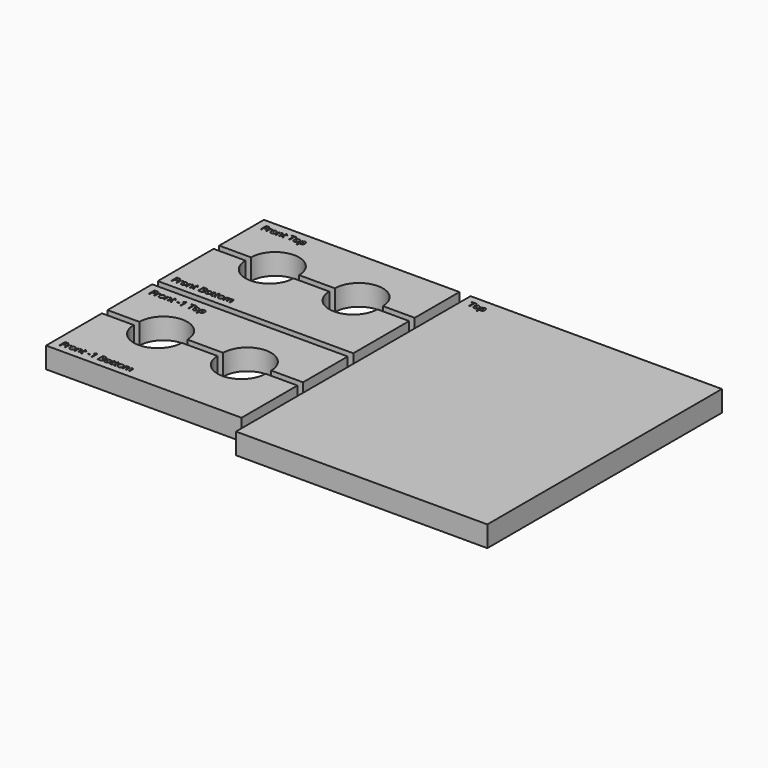
from build123d import *

# Parameters (mm, degrees)
F1_DEPTH = 9.525
F0_W     = 1.0569552951
F0_H     = 0.3272840712
F0_W_2   = 114.3
F0_H_2   = 133.35


# Not quite as in the source:
# - a length typed as a fraction of an inch, garbled in the dataset ("3 / 203.2 mm" for 3/8 in), is restored


with BuildPart() as f1:
    # F0 (on Top) → F1 (new body)
    with BuildSketch(Plane.XY):
        with BuildLine():
            Line((44.45, 0), (-44.45, 0))
            Line((-44.45, 0), (-44.45, -25.4))
            Line((-44.45, -25.4), (-29.972, -25.4))
            ThreePointArc((-29.972, -25.4), (-19.05, -14.478), (-8.128, -25.4))
            Line((-8.128, -25.4), (8.128, -25.4))
            ThreePointArc((8.128, -25.4), (19.05, -14.478), (29.972, -25.4))
            Line((29.972, -25.4), (44.45, -25.4))
            Line((44.45, -25.4), (44.45, 0))
        make_face()
        Polygon((-40.4764268663, -5.0043457031), (-40.4764268663, -6.35), (-40.8422960069, -6.35), (-40.8422960069, -3.2018717448), (-39.0873643663, -3.2018717448), (-39.0873643663, -3.5270887587), (-40.4764268663, -3.5270887587), (-40.4764268663, -4.6791286892), (-39.1714246962, -4.6791286892), (-39.1714246962, -5.0043457031), align=None, mode=Mode.SUBTRACT)
        with BuildLine():
            add(Edge.make_bspline(
                [(-37.9504828559, -4.071758355), (-37.7651367187, -3.9467013889), (-37.5432725694, -3.9467013889)],
                knots=[0, 0, 0, 1, 1, 1], degree=2))
            add(Edge.make_bspline(
                [(-37.5432725694, -3.9467013889), (-37.3861762153, -3.9467013889), (-37.2614637587, -3.9728841146)],
                knots=[0, 0, 0, 1, 1, 1], degree=2))
            Line((-37.2614637587, -3.9728841146), (-37.3110731337, -4.3043023003))
            add(Edge.make_bspline(
                [(-37.3110731337, -4.3043023003), (-37.4571451823, -4.2719184028), (-37.5694552951, -4.2719184028)],
                knots=[0, 0, 0, 1, 1, 1], degree=2))
            add(Edge.make_bspline(
                [(-37.5694552951, -4.2719184028), (-37.8560872396, -4.2719184028), (-38.0593478733, -4.5044623481)],
                knots=[0, 0, 0, 1, 1, 1], degree=2))
            add(Edge.make_bspline(
                [(-38.0593478733, -4.5044623481), (-38.2626085069, -4.7370062934), (-38.2626085069, -5.0835828993)],
                knots=[0, 0, 0, 1, 1, 1], degree=2))
            Line((-38.2626085069, -5.0835828993), (-38.2626085069, -6.35))
            Line((-38.2626085069, -6.35), (-38.6202094184, -6.35))
            Line((-38.6202094184, -6.35), (-38.6202094184, -3.990109592))
            Line((-38.6202094184, -3.990109592), (-38.3253092448, -3.990109592))
            Line((-38.3253092448, -3.990109592), (-38.283968099, -4.4269476997))
            Line((-38.283968099, -4.4269476997), (-38.2667426215, -4.4269476997))
            add(Edge.make_bspline(
                [(-38.2667426215, -4.4269476997), (-38.1358289931, -4.1968153212), (-37.9504828559, -4.071758355)],
                knots=[0, 0, 0, 1, 1, 1], degree=2))
        make_face(mode=Mode.SUBTRACT)
        with BuildLine():
            add(Edge.make_bspline(
                [(-35.0748616536, -4.2763970269), (-34.783062066, -4.6060926649), (-34.783062066, -5.1676432292)],
                knots=[0, 0, 0, 1, 1, 1], degree=2))
            add(Edge.make_bspline(
                [(-34.783062066, -5.1676432292), (-34.783062066, -5.7450412326), (-35.0734836155, -6.0692247179)],
                knots=[0, 0, 0, 1, 1, 1], degree=2))
            add(Edge.make_bspline(
                [(-35.0734836155, -6.0692247179), (-35.3639051649, -6.3934082031), (-35.8765353733, -6.3934082031)],
                knots=[0, 0, 0, 1, 1, 1], degree=2))
            add(Edge.make_bspline(
                [(-35.8765353733, -6.3934082031), (-36.193484158, -6.3934082031), (-36.4387749566, -6.2445800781)],
                knots=[0, 0, 0, 1, 1, 1], degree=2))
            add(Edge.make_bspline(
                [(-36.4387749566, -6.2445800781), (-36.6840657552, -6.0957519531), (-36.8177354601, -5.8180772569)],
                knots=[0, 0, 0, 1, 1, 1], degree=2))
            add(Edge.make_bspline(
                [(-36.8177354601, -5.8180772569), (-36.9514051649, -5.5404025608), (-36.9514051649, -5.1676432292)],
                knots=[0, 0, 0, 1, 1, 1], degree=2))
            add(Edge.make_bspline(
                [(-36.9514051649, -5.1676432292), (-36.9514051649, -4.5909342448), (-36.6627061632, -4.2688178168)],
                knots=[0, 0, 0, 1, 1, 1], degree=2))
            add(Edge.make_bspline(
                [(-36.6627061632, -4.2688178168), (-36.3740071615, -3.9467013889), (-35.8613769531, -3.9467013889)],
                knots=[0, 0, 0, 1, 1, 1], degree=2))
            add(Edge.make_bspline(
                [(-35.8613769531, -3.9467013889), (-35.3666612413, -3.9467013889), (-35.0748616536, -4.2763970269)],
                knots=[0, 0, 0, 1, 1, 1], degree=2))
        make_face(mode=Mode.SUBTRACT)
        with BuildLine():
            Line((-32.1833930122, -6.35), (-32.5409939236, -6.35))
            Line((-32.5409939236, -6.35), (-32.5409939236, -4.8231336806))
            add(Edge.make_bspline(
                [(-32.5409939236, -4.8231336806), (-32.5409939236, -4.5351236979), (-32.6722520616, -4.3928412543)],
                knots=[0, 0, 0, 1, 1, 1], degree=2))
            add(Edge.make_bspline(
                [(-32.6722520616, -4.3928412543), (-32.8035101997, -4.2505588108), (-33.0839409722, -4.2505588108)],
                knots=[0, 0, 0, 1, 1, 1], degree=2))
            add(Edge.make_bspline(
                [(-33.0839409722, -4.2505588108), (-33.4539442274, -4.2505588108), (-33.6261990017, -4.4507188585)],
                knots=[0, 0, 0, 1, 1, 1], degree=2))
            add(Edge.make_bspline(
                [(-33.6261990017, -4.4507188585), (-33.798453776, -4.6508789062), (-33.798453776, -5.1118326823)],
                knots=[0, 0, 0, 1, 1, 1], degree=2))
            Line((-33.798453776, -5.1118326823), (-33.798453776, -6.35))
            Line((-33.798453776, -6.35), (-34.1560546875, -6.35))
            Line((-34.1560546875, -6.35), (-34.1560546875, -3.990109592))
            Line((-34.1560546875, -3.990109592), (-33.8652886285, -3.990109592))
            Line((-33.8652886285, -3.990109592), (-33.8074110243, -4.3132595486))
            Line((-33.8074110243, -4.3132595486), (-33.7901855469, -4.3132595486))
            add(Edge.make_bspline(
                [(-33.7901855469, -4.3132595486), (-33.6799424913, -4.138937717), (-33.4818495009, -4.042819553)],
                knots=[0, 0, 0, 1, 1, 1], degree=2))
            add(Edge.make_bspline(
                [(-33.4818495009, -4.042819553), (-33.2837565104, -3.9467013889), (-33.0405327691, -3.9467013889)],
                knots=[0, 0, 0, 1, 1, 1], degree=2))
            add(Edge.make_bspline(
                [(-33.0405327691, -3.9467013889), (-32.6140299479, -3.9467013889), (-32.39871148, -4.1523735894)],
                knots=[0, 0, 0, 1, 1, 1], degree=2))
            add(Edge.make_bspline(
                [(-32.39871148, -4.1523735894), (-32.1833930122, -4.3580457899), (-32.1833930122, -4.8107313368)],
                knots=[0, 0, 0, 1, 1, 1], degree=2))
            Line((-32.1833930122, -4.8107313368), (-32.1833930122, -6.35))
        make_face(mode=Mode.SUBTRACT)
        with BuildLine():
            add(Edge.make_bspline(
                [(-30.9652072483, -5.9837863498), (-30.863921441, -6.0978190104), (-30.6875325521, -6.0978190104)],
                knots=[0, 0, 0, 1, 1, 1], degree=2))
            add(Edge.make_bspline(
                [(-30.6875325521, -6.0978190104), (-30.5924479167, -6.0978190104), (-30.5042534722, -6.0840386285)],
                knots=[0, 0, 0, 1, 1, 1], degree=2))
            add(Edge.make_bspline(
                [(-30.5042534722, -6.0840386285), (-30.4160590278, -6.0702582465), (-30.3643825955, -6.0550998264)],
                knots=[0, 0, 0, 1, 1, 1], degree=2))
            Line((-30.3643825955, -6.0550998264), (-30.3643825955, -6.328640408))
            add(Edge.make_bspline(
                [(-30.3643825955, -6.328640408), (-30.4222601997, -6.3562011719), (-30.5352593316, -6.3748046875)],
                knots=[0, 0, 0, 1, 1, 1], degree=2))
            add(Edge.make_bspline(
                [(-30.5352593316, -6.3748046875), (-30.6482584635, -6.3934082031), (-30.7392089844, -6.3934082031)],
                knots=[0, 0, 0, 1, 1, 1], degree=2))
            add(Edge.make_bspline(
                [(-30.7392089844, -6.3934082031), (-31.4234049479, -6.3934082031), (-31.4234049479, -5.6720052083)],
                knots=[0, 0, 0, 1, 1, 1], degree=2))
            Line((-31.4234049479, -5.6720052083), (-31.4234049479, -4.2677842882))
            Line((-31.4234049479, -4.2677842882), (-31.7617133247, -4.2677842882))
            Line((-31.7617133247, -4.2677842882), (-31.7617133247, -4.0955295139))
            Line((-31.7617133247, -4.0955295139), (-31.4234049479, -3.9467013889))
            Line((-31.4234049479, -3.9467013889), (-31.2731987847, -3.4430284288))
            Line((-31.2731987847, -3.4430284288), (-31.0664930556, -3.4430284288))
            Line((-31.0664930556, -3.4430284288), (-31.0664930556, -3.990109592))
            Line((-31.0664930556, -3.990109592), (-30.3816080729, -3.990109592))
            Line((-30.3816080729, -3.990109592), (-30.3816080729, -4.2677842882))
            Line((-30.3816080729, -4.2677842882), (-31.0664930556, -4.2677842882))
            Line((-31.0664930556, -4.2677842882), (-31.0664930556, -5.6568467882))
            add(Edge.make_bspline(
                [(-31.0664930556, -5.6568467882), (-31.0664930556, -5.8697536892), (-30.9652072483, -5.9837863498)],
                knots=[0, 0, 0, 1, 1, 1], degree=2))
        make_face(mode=Mode.SUBTRACT)
        Polygon((-27.724750434, -3.5270887587), (-27.724750434, -6.35), (-28.0906195747, -6.35), (-28.0906195747, -3.5270887587), (-29.0876302083, -3.5270887587), (-29.0876302083, -3.2018717448), (-26.7277398003, -3.2018717448), (-26.7277398003, -3.5270887587), align=None, mode=Mode.SUBTRACT)
        with BuildLine():
            add(Edge.make_bspline(
                [(-24.5624972873, -4.2763970269), (-24.2706976997, -4.6060926649), (-24.2706976997, -5.1676432292)],
                knots=[0, 0, 0, 1, 1, 1], degree=2))
            add(Edge.make_bspline(
                [(-24.2706976997, -5.1676432292), (-24.2706976997, -5.7450412326), (-24.5611192491, -6.0692247179)],
                knots=[0, 0, 0, 1, 1, 1], degree=2))
            add(Edge.make_bspline(
                [(-24.5611192491, -6.0692247179), (-24.8515407986, -6.3934082031), (-25.3641710069, -6.3934082031)],
                knots=[0, 0, 0, 1, 1, 1], degree=2))
            add(Edge.make_bspline(
                [(-25.3641710069, -6.3934082031), (-25.6811197917, -6.3934082031), (-25.9264105903, -6.2445800781)],
                knots=[0, 0, 0, 1, 1, 1], degree=2))
            add(Edge.make_bspline(
                [(-25.9264105903, -6.2445800781), (-26.1717013889, -6.0957519531), (-26.3053710937, -5.8180772569)],
                knots=[0, 0, 0, 1, 1, 1], degree=2))
            add(Edge.make_bspline(
                [(-26.3053710937, -5.8180772569), (-26.4390407986, -5.5404025608), (-26.4390407986, -5.1676432292)],
                knots=[0, 0, 0, 1, 1, 1], degree=2))
            add(Edge.make_bspline(
                [(-26.4390407986, -5.1676432292), (-26.4390407986, -4.5909342448), (-26.1503417969, -4.2688178168)],
                knots=[0, 0, 0, 1, 1, 1], degree=2))
            add(Edge.make_bspline(
                [(-26.1503417969, -4.2688178168), (-25.8616427951, -3.9467013889), (-25.3490125868, -3.9467013889)],
                knots=[0, 0, 0, 1, 1, 1], degree=2))
            add(Edge.make_bspline(
                [(-25.3490125868, -3.9467013889), (-24.854296875, -3.9467013889), (-24.5624972873, -4.2763970269)],
                knots=[0, 0, 0, 1, 1, 1], degree=2))
        make_face(mode=Mode.SUBTRACT)
        with BuildLine():
            add(Edge.make_bspline(
                [(-21.8250244141, -6.0712917752), (-22.0844401042, -6.3934082031), (-22.5453938802, -6.3934082031)],
                knots=[0, 0, 0, 1, 1, 1], degree=2))
            add(Edge.make_bspline(
                [(-22.5453938802, -6.3934082031), (-22.7762152778, -6.3934082031), (-22.9667290582, -6.3083143446)],
                knots=[0, 0, 0, 1, 1, 1], degree=2))
            add(Edge.make_bspline(
                [(-22.9667290582, -6.3083143446), (-23.1572428385, -6.2232204861), (-23.2860894097, -6.0461425781)],
                knots=[0, 0, 0, 1, 1, 1], degree=2))
            Line((-23.2860894097, -6.0461425781), (-23.3122721354, -6.0461425781))
            add(Edge.make_bspline(
                [(-23.3122721354, -6.0461425781), (-23.2860894097, -6.2528483073), (-23.2860894097, -6.4381944444)],
                knots=[0, 0, 0, 1, 1, 1], degree=2))
            Line((-23.2860894097, -6.4381944444), (-23.2860894097, -7.4097113715))
            Line((-23.2860894097, -7.4097113715), (-23.6436903212, -7.4097113715))
            Line((-23.6436903212, -7.4097113715), (-23.6436903212, -3.990109592))
            Line((-23.6436903212, -3.990109592), (-23.3529242622, -3.990109592))
            Line((-23.3529242622, -3.990109592), (-23.3033148872, -4.3132595486))
            Line((-23.3033148872, -4.3132595486), (-23.2860894097, -4.3132595486))
            add(Edge.make_bspline(
                [(-23.2860894097, -4.3132595486), (-23.1482855903, -4.1189561632), (-22.96535102, -4.032828776)],
                knots=[0, 0, 0, 1, 1, 1], degree=2))
            add(Edge.make_bspline(
                [(-22.96535102, -4.032828776), (-22.7824164497, -3.9467013889), (-22.5453938802, -3.9467013889)],
                knots=[0, 0, 0, 1, 1, 1], degree=2))
            add(Edge.make_bspline(
                [(-22.5453938802, -3.9467013889), (-22.076171875, -3.9467013889), (-21.8208902995, -4.2677842882)],
                knots=[0, 0, 0, 1, 1, 1], degree=2))
            add(Edge.make_bspline(
                [(-21.8208902995, -4.2677842882), (-21.565608724, -4.5888671875), (-21.565608724, -5.1676432292)],
                knots=[0, 0, 0, 1, 1, 1], degree=2))
            add(Edge.make_bspline(
                [(-21.565608724, -5.1676432292), (-21.565608724, -5.7491753472), (-21.8250244141, -6.0712917752)],
                knots=[0, 0, 0, 1, 1, 1], degree=2))
        make_face(mode=Mode.SUBTRACT)
    extrude(amount=F1_DEPTH)


with BuildPart() as f1b:
    # F0 (on Top) → F1, piece 2 (new body)
    with BuildSketch(Plane.XY):
        with BuildLine():
            Line((-29.972, -28.575), (-44.45, -28.575))
            Line((-44.45, -28.575), (-44.45, -60.325))
            Line((-44.45, -60.325), (44.45, -60.325))
            Line((44.45, -60.325), (44.45, -28.575))
            Line((44.45, -28.575), (29.972, -28.575))
            ThreePointArc((29.972, -28.575), (19.05, -39.497), (8.128, -28.575))
            Line((8.128, -28.575), (-8.128, -28.575))
            ThreePointArc((-8.128, -28.575), (-19.05, -39.497), (-29.972, -28.575))
        make_face()
        Polygon((-40.4764268663, -55.8043457031), (-40.4764268663, -57.15), (-40.8422960069, -57.15), (-40.8422960069, -54.0018717448), (-39.0873643663, -54.0018717448), (-39.0873643663, -54.3270887587), (-40.4764268663, -54.3270887587), (-40.4764268663, -55.4791286892), (-39.1714246962, -55.4791286892), (-39.1714246962, -55.8043457031), align=None, mode=Mode.SUBTRACT)
        with BuildLine():
            add(Edge.make_bspline(
                [(-37.9504828559, -54.871758355), (-37.7651367187, -54.7467013889), (-37.5432725694, -54.7467013889)],
                knots=[0, 0, 0, 1, 1, 1], degree=2))
            add(Edge.make_bspline(
                [(-37.5432725694, -54.7467013889), (-37.3861762153, -54.7467013889), (-37.2614637587, -54.7728841146)],
                knots=[0, 0, 0, 1, 1, 1], degree=2))
            Line((-37.2614637587, -54.7728841146), (-37.3110731337, -55.1043023003))
            add(Edge.make_bspline(
                [(-37.3110731337, -55.1043023003), (-37.4571451823, -55.0719184028), (-37.5694552951, -55.0719184028)],
                knots=[0, 0, 0, 1, 1, 1], degree=2))
            add(Edge.make_bspline(
                [(-37.5694552951, -55.0719184028), (-37.8560872396, -55.0719184028), (-38.0593478733, -55.3044623481)],
                knots=[0, 0, 0, 1, 1, 1], degree=2))
            add(Edge.make_bspline(
                [(-38.0593478733, -55.3044623481), (-38.2626085069, -55.5370062934), (-38.2626085069, -55.8835828993)],
                knots=[0, 0, 0, 1, 1, 1], degree=2))
            Line((-38.2626085069, -55.8835828993), (-38.2626085069, -57.15))
            Line((-38.2626085069, -57.15), (-38.6202094184, -57.15))
            Line((-38.6202094184, -57.15), (-38.6202094184, -54.790109592))
            Line((-38.6202094184, -54.790109592), (-38.3253092448, -54.790109592))
            Line((-38.3253092448, -54.790109592), (-38.283968099, -55.2269476997))
            Line((-38.283968099, -55.2269476997), (-38.2667426215, -55.2269476997))
            add(Edge.make_bspline(
                [(-38.2667426215, -55.2269476997), (-38.1358289931, -54.9968153212), (-37.9504828559, -54.871758355)],
                knots=[0, 0, 0, 1, 1, 1], degree=2))
        make_face(mode=Mode.SUBTRACT)
        with BuildLine():
            add(Edge.make_bspline(
                [(-35.0748616536, -55.0763970269), (-34.783062066, -55.4060926649), (-34.783062066, -55.9676432292)],
                knots=[0, 0, 0, 1, 1, 1], degree=2))
            add(Edge.make_bspline(
                [(-34.783062066, -55.9676432292), (-34.783062066, -56.5450412326), (-35.0734836155, -56.8692247179)],
                knots=[0, 0, 0, 1, 1, 1], degree=2))
            add(Edge.make_bspline(
                [(-35.0734836155, -56.8692247179), (-35.3639051649, -57.1934082031), (-35.8765353733, -57.1934082031)],
                knots=[0, 0, 0, 1, 1, 1], degree=2))
            add(Edge.make_bspline(
                [(-35.8765353733, -57.1934082031), (-36.193484158, -57.1934082031), (-36.4387749566, -57.0445800781)],
                knots=[0, 0, 0, 1, 1, 1], degree=2))
            add(Edge.make_bspline(
                [(-36.4387749566, -57.0445800781), (-36.6840657552, -56.8957519531), (-36.8177354601, -56.6180772569)],
                knots=[0, 0, 0, 1, 1, 1], degree=2))
            add(Edge.make_bspline(
                [(-36.8177354601, -56.6180772569), (-36.9514051649, -56.3404025608), (-36.9514051649, -55.9676432292)],
                knots=[0, 0, 0, 1, 1, 1], degree=2))
            add(Edge.make_bspline(
                [(-36.9514051649, -55.9676432292), (-36.9514051649, -55.3909342448), (-36.6627061632, -55.0688178168)],
                knots=[0, 0, 0, 1, 1, 1], degree=2))
            add(Edge.make_bspline(
                [(-36.6627061632, -55.0688178168), (-36.3740071615, -54.7467013889), (-35.8613769531, -54.7467013889)],
                knots=[0, 0, 0, 1, 1, 1], degree=2))
            add(Edge.make_bspline(
                [(-35.8613769531, -54.7467013889), (-35.3666612413, -54.7467013889), (-35.0748616536, -55.0763970269)],
                knots=[0, 0, 0, 1, 1, 1], degree=2))
        make_face(mode=Mode.SUBTRACT)
        with BuildLine():
            Line((-32.1833930122, -57.15), (-32.5409939236, -57.15))
            Line((-32.5409939236, -57.15), (-32.5409939236, -55.6231336806))
            add(Edge.make_bspline(
                [(-32.5409939236, -55.6231336806), (-32.5409939236, -55.3351236979), (-32.6722520616, -55.1928412543)],
                knots=[0, 0, 0, 1, 1, 1], degree=2))
            add(Edge.make_bspline(
                [(-32.6722520616, -55.1928412543), (-32.8035101997, -55.0505588108), (-33.0839409722, -55.0505588108)],
                knots=[0, 0, 0, 1, 1, 1], degree=2))
            add(Edge.make_bspline(
                [(-33.0839409722, -55.0505588108), (-33.4539442274, -55.0505588108), (-33.6261990017, -55.2507188585)],
                knots=[0, 0, 0, 1, 1, 1], degree=2))
            add(Edge.make_bspline(
                [(-33.6261990017, -55.2507188585), (-33.798453776, -55.4508789062), (-33.798453776, -55.9118326823)],
                knots=[0, 0, 0, 1, 1, 1], degree=2))
            Line((-33.798453776, -55.9118326823), (-33.798453776, -57.15))
            Line((-33.798453776, -57.15), (-34.1560546875, -57.15))
            Line((-34.1560546875, -57.15), (-34.1560546875, -54.790109592))
            Line((-34.1560546875, -54.790109592), (-33.8652886285, -54.790109592))
            Line((-33.8652886285, -54.790109592), (-33.8074110243, -55.1132595486))
            Line((-33.8074110243, -55.1132595486), (-33.7901855469, -55.1132595486))
            add(Edge.make_bspline(
                [(-33.7901855469, -55.1132595486), (-33.6799424913, -54.938937717), (-33.4818495009, -54.842819553)],
                knots=[0, 0, 0, 1, 1, 1], degree=2))
            add(Edge.make_bspline(
                [(-33.4818495009, -54.842819553), (-33.2837565104, -54.7467013889), (-33.0405327691, -54.7467013889)],
                knots=[0, 0, 0, 1, 1, 1], degree=2))
            add(Edge.make_bspline(
                [(-33.0405327691, -54.7467013889), (-32.6140299479, -54.7467013889), (-32.39871148, -54.9523735894)],
                knots=[0, 0, 0, 1, 1, 1], degree=2))
            add(Edge.make_bspline(
                [(-32.39871148, -54.9523735894), (-32.1833930122, -55.1580457899), (-32.1833930122, -55.6107313368)],
                knots=[0, 0, 0, 1, 1, 1], degree=2))
            Line((-32.1833930122, -55.6107313368), (-32.1833930122, -57.15))
        make_face(mode=Mode.SUBTRACT)
        with BuildLine():
            add(Edge.make_bspline(
                [(-30.9652072483, -56.7837863498), (-30.863921441, -56.8978190104), (-30.6875325521, -56.8978190104)],
                knots=[0, 0, 0, 1, 1, 1], degree=2))
            add(Edge.make_bspline(
                [(-30.6875325521, -56.8978190104), (-30.5924479167, -56.8978190104), (-30.5042534722, -56.8840386285)],
                knots=[0, 0, 0, 1, 1, 1], degree=2))
            add(Edge.make_bspline(
                [(-30.5042534722, -56.8840386285), (-30.4160590278, -56.8702582465), (-30.3643825955, -56.8550998264)],
                knots=[0, 0, 0, 1, 1, 1], degree=2))
            Line((-30.3643825955, -56.8550998264), (-30.3643825955, -57.128640408))
            add(Edge.make_bspline(
                [(-30.3643825955, -57.128640408), (-30.4222601997, -57.1562011719), (-30.5352593316, -57.1748046875)],
                knots=[0, 0, 0, 1, 1, 1], degree=2))
            add(Edge.make_bspline(
                [(-30.5352593316, -57.1748046875), (-30.6482584635, -57.1934082031), (-30.7392089844, -57.1934082031)],
                knots=[0, 0, 0, 1, 1, 1], degree=2))
            add(Edge.make_bspline(
                [(-30.7392089844, -57.1934082031), (-31.4234049479, -57.1934082031), (-31.4234049479, -56.4720052083)],
                knots=[0, 0, 0, 1, 1, 1], degree=2))
            Line((-31.4234049479, -56.4720052083), (-31.4234049479, -55.0677842882))
            Line((-31.4234049479, -55.0677842882), (-31.7617133247, -55.0677842882))
            Line((-31.7617133247, -55.0677842882), (-31.7617133247, -54.8955295139))
            Line((-31.7617133247, -54.8955295139), (-31.4234049479, -54.7467013889))
            Line((-31.4234049479, -54.7467013889), (-31.2731987847, -54.2430284288))
            Line((-31.2731987847, -54.2430284288), (-31.0664930556, -54.2430284288))
            Line((-31.0664930556, -54.2430284288), (-31.0664930556, -54.790109592))
            Line((-31.0664930556, -54.790109592), (-30.3816080729, -54.790109592))
            Line((-30.3816080729, -54.790109592), (-30.3816080729, -55.0677842882))
            Line((-30.3816080729, -55.0677842882), (-31.0664930556, -55.0677842882))
            Line((-31.0664930556, -55.0677842882), (-31.0664930556, -56.4568467882))
            add(Edge.make_bspline(
                [(-31.0664930556, -56.4568467882), (-31.0664930556, -56.6697536892), (-30.9652072483, -56.7837863498)],
                knots=[0, 0, 0, 1, 1, 1], degree=2))
        make_face(mode=Mode.SUBTRACT)
        with BuildLine():
            Line((-28.6935112847, -57.15), (-28.6935112847, -54.0018717448))
            Line((-28.6935112847, -54.0018717448), (-27.8039876302, -54.0018717448))
            add(Edge.make_bspline(
                [(-27.8039876302, -54.0018717448), (-27.1776692708, -54.0018717448), (-26.8975830078, -54.1892849392)],
                knots=[0, 0, 0, 1, 1, 1], degree=2))
            add(Edge.make_bspline(
                [(-26.8975830078, -54.1892849392), (-26.6174967448, -54.3766981337), (-26.6174967448, -54.7811523437)],
                knots=[0, 0, 0, 1, 1, 1], degree=2))
            add(Edge.make_bspline(
                [(-26.6174967448, -54.7811523437), (-26.6174967448, -55.0615831163), (-26.7735595703, -55.243484158)],
                knots=[0, 0, 0, 1, 1, 1], degree=2))
            add(Edge.make_bspline(
                [(-26.7735595703, -55.243484158), (-26.9296223958, -55.4253851997), (-27.2293457031, -55.4791286892)],
                knots=[0, 0, 0, 1, 1, 1], degree=2))
            Line((-27.2293457031, -55.4791286892), (-27.2293457031, -55.5004882812))
            add(Edge.make_bspline(
                [(-27.2293457031, -55.5004882812), (-26.5120768229, -55.6231336806), (-26.5120768229, -56.2542751736)],
                knots=[0, 0, 0, 1, 1, 1], degree=2))
            add(Edge.make_bspline(
                [(-26.5120768229, -56.2542751736), (-26.5120768229, -56.6759548611), (-26.7973307292, -56.9129774306)],
                knots=[0, 0, 0, 1, 1, 1], degree=2))
            add(Edge.make_bspline(
                [(-26.7973307292, -56.9129774306), (-27.0825846354, -57.15), (-27.5952148437, -57.15)],
                knots=[0, 0, 0, 1, 1, 1], degree=2))
            Line((-27.5952148437, -57.15), (-28.6935112847, -57.15))
        make_face(mode=Mode.SUBTRACT)
        with BuildLine():
            add(Edge.make_bspline(
                [(-24.1449517144, -55.0763970269), (-23.8531521267, -55.4060926649), (-23.8531521267, -55.9676432292)],
                knots=[0, 0, 0, 1, 1, 1], degree=2))
            add(Edge.make_bspline(
                [(-23.8531521267, -55.9676432292), (-23.8531521267, -56.5450412326), (-24.1435736762, -56.8692247179)],
                knots=[0, 0, 0, 1, 1, 1], degree=2))
            add(Edge.make_bspline(
                [(-24.1435736762, -56.8692247179), (-24.4339952257, -57.1934082031), (-24.946625434, -57.1934082031)],
                knots=[0, 0, 0, 1, 1, 1], degree=2))
            add(Edge.make_bspline(
                [(-24.946625434, -57.1934082031), (-25.2635742187, -57.1934082031), (-25.5088650174, -57.0445800781)],
                knots=[0, 0, 0, 1, 1, 1], degree=2))
            add(Edge.make_bspline(
                [(-25.5088650174, -57.0445800781), (-25.754155816, -56.8957519531), (-25.8878255208, -56.6180772569)],
                knots=[0, 0, 0, 1, 1, 1], degree=2))
            add(Edge.make_bspline(
                [(-25.8878255208, -56.6180772569), (-26.0214952257, -56.3404025608), (-26.0214952257, -55.9676432292)],
                knots=[0, 0, 0, 1, 1, 1], degree=2))
            add(Edge.make_bspline(
                [(-26.0214952257, -55.9676432292), (-26.0214952257, -55.3909342448), (-25.732796224, -55.0688178168)],
                knots=[0, 0, 0, 1, 1, 1], degree=2))
            add(Edge.make_bspline(
                [(-25.732796224, -55.0688178168), (-25.4440972222, -54.7467013889), (-24.9314670139, -54.7467013889)],
                knots=[0, 0, 0, 1, 1, 1], degree=2))
            add(Edge.make_bspline(
                [(-24.9314670139, -54.7467013889), (-24.4367513021, -54.7467013889), (-24.1449517144, -55.0763970269)],
                knots=[0, 0, 0, 1, 1, 1], degree=2))
        make_face(mode=Mode.SUBTRACT)
        with BuildLine():
            add(Edge.make_bspline(
                [(-22.7417643229, -56.7837863498), (-22.6404785156, -56.8978190104), (-22.4640896267, -56.8978190104)],
                knots=[0, 0, 0, 1, 1, 1], degree=2))
            add(Edge.make_bspline(
                [(-22.4640896267, -56.8978190104), (-22.3690049913, -56.8978190104), (-22.2808105469, -56.8840386285)],
                knots=[0, 0, 0, 1, 1, 1], degree=2))
            add(Edge.make_bspline(
                [(-22.2808105469, -56.8840386285), (-22.1926161024, -56.8702582465), (-22.1409396701, -56.8550998264)],
                knots=[0, 0, 0, 1, 1, 1], degree=2))
            Line((-22.1409396701, -56.8550998264), (-22.1409396701, -57.128640408))
            add(Edge.make_bspline(
                [(-22.1409396701, -57.128640408), (-22.1988172743, -57.1562011719), (-22.3118164062, -57.1748046875)],
                knots=[0, 0, 0, 1, 1, 1], degree=2))
            add(Edge.make_bspline(
                [(-22.3118164062, -57.1748046875), (-22.4248155382, -57.1934082031), (-22.515766059, -57.1934082031)],
                knots=[0, 0, 0, 1, 1, 1], degree=2))
            add(Edge.make_bspline(
                [(-22.515766059, -57.1934082031), (-23.1999620226, -57.1934082031), (-23.1999620226, -56.4720052083)],
                knots=[0, 0, 0, 1, 1, 1], degree=2))
            Line((-23.1999620226, -56.4720052083), (-23.1999620226, -55.0677842882))
            Line((-23.1999620226, -55.0677842882), (-23.5382703993, -55.0677842882))
            Line((-23.5382703993, -55.0677842882), (-23.5382703993, -54.8955295139))
            Line((-23.5382703993, -54.8955295139), (-23.1999620226, -54.7467013889))
            Line((-23.1999620226, -54.7467013889), (-23.0497558594, -54.2430284288))
            Line((-23.0497558594, -54.2430284288), (-22.8430501302, -54.2430284288))
            Line((-22.8430501302, -54.2430284288), (-22.8430501302, -54.790109592))
            Line((-22.8430501302, -54.790109592), (-22.1581651476, -54.790109592))
            Line((-22.1581651476, -54.790109592), (-22.1581651476, -55.0677842882))
            Line((-22.1581651476, -55.0677842882), (-22.8430501302, -55.0677842882))
            Line((-22.8430501302, -55.0677842882), (-22.8430501302, -56.4568467882))
            add(Edge.make_bspline(
                [(-22.8430501302, -56.4568467882), (-22.8430501302, -56.6697536892), (-22.7417643229, -56.7837863498)],
                knots=[0, 0, 0, 1, 1, 1], degree=2))
        make_face(mode=Mode.SUBTRACT)
        with BuildLine():
            add(Edge.make_bspline(
                [(-21.1852701823, -56.7837863498), (-21.083984375, -56.8978190104), (-20.9075954861, -56.8978190104)],
                knots=[0, 0, 0, 1, 1, 1], degree=2))
            add(Edge.make_bspline(
                [(-20.9075954861, -56.8978190104), (-20.8125108507, -56.8978190104), (-20.7243164062, -56.8840386285)],
                knots=[0, 0, 0, 1, 1, 1], degree=2))
            add(Edge.make_bspline(
                [(-20.7243164062, -56.8840386285), (-20.6361219618, -56.8702582465), (-20.5844455295, -56.8550998264)],
                knots=[0, 0, 0, 1, 1, 1], degree=2))
            Line((-20.5844455295, -56.8550998264), (-20.5844455295, -57.128640408))
            add(Edge.make_bspline(
                [(-20.5844455295, -57.128640408), (-20.6423231337, -57.1562011719), (-20.7553222656, -57.1748046875)],
                knots=[0, 0, 0, 1, 1, 1], degree=2))
            add(Edge.make_bspline(
                [(-20.7553222656, -57.1748046875), (-20.8683213976, -57.1934082031), (-20.9592719184, -57.1934082031)],
                knots=[0, 0, 0, 1, 1, 1], degree=2))
            add(Edge.make_bspline(
                [(-20.9592719184, -57.1934082031), (-21.6434678819, -57.1934082031), (-21.6434678819, -56.4720052083)],
                knots=[0, 0, 0, 1, 1, 1], degree=2))
            Line((-21.6434678819, -56.4720052083), (-21.6434678819, -55.0677842882))
            Line((-21.6434678819, -55.0677842882), (-21.9817762587, -55.0677842882))
            Line((-21.9817762587, -55.0677842882), (-21.9817762587, -54.8955295139))
            Line((-21.9817762587, -54.8955295139), (-21.6434678819, -54.7467013889))
            Line((-21.6434678819, -54.7467013889), (-21.4932617187, -54.2430284288))
            Line((-21.4932617187, -54.2430284288), (-21.2865559896, -54.2430284288))
            Line((-21.2865559896, -54.2430284288), (-21.2865559896, -54.790109592))
            Line((-21.2865559896, -54.790109592), (-20.6016710069, -54.790109592))
            Line((-20.6016710069, -54.790109592), (-20.6016710069, -55.0677842882))
            Line((-20.6016710069, -55.0677842882), (-21.2865559896, -55.0677842882))
            Line((-21.2865559896, -55.0677842882), (-21.2865559896, -56.4568467882))
            add(Edge.make_bspline(
                [(-21.2865559896, -56.4568467882), (-21.2865559896, -56.6697536892), (-21.1852701823, -56.7837863498)],
                knots=[0, 0, 0, 1, 1, 1], degree=2))
        make_face(mode=Mode.SUBTRACT)
        with BuildLine():
            add(Edge.make_bspline(
                [(-18.3682156033, -55.0763970269), (-18.0764160156, -55.4060926649), (-18.0764160156, -55.9676432292)],
                knots=[0, 0, 0, 1, 1, 1], degree=2))
            add(Edge.make_bspline(
                [(-18.0764160156, -55.9676432292), (-18.0764160156, -56.5450412326), (-18.3668375651, -56.8692247179)],
                knots=[0, 0, 0, 1, 1, 1], degree=2))
            add(Edge.make_bspline(
                [(-18.3668375651, -56.8692247179), (-18.6572591146, -57.1934082031), (-19.1698893229, -57.1934082031)],
                knots=[0, 0, 0, 1, 1, 1], degree=2))
            add(Edge.make_bspline(
                [(-19.1698893229, -57.1934082031), (-19.4868381076, -57.1934082031), (-19.7321289062, -57.0445800781)],
                knots=[0, 0, 0, 1, 1, 1], degree=2))
            add(Edge.make_bspline(
                [(-19.7321289062, -57.0445800781), (-19.9774197049, -56.8957519531), (-20.1110894097, -56.6180772569)],
                knots=[0, 0, 0, 1, 1, 1], degree=2))
            add(Edge.make_bspline(
                [(-20.1110894097, -56.6180772569), (-20.2447591146, -56.3404025608), (-20.2447591146, -55.9676432292)],
                knots=[0, 0, 0, 1, 1, 1], degree=2))
            add(Edge.make_bspline(
                [(-20.2447591146, -55.9676432292), (-20.2447591146, -55.3909342448), (-19.9560601128, -55.0688178168)],
                knots=[0, 0, 0, 1, 1, 1], degree=2))
            add(Edge.make_bspline(
                [(-19.9560601128, -55.0688178168), (-19.6673611111, -54.7467013889), (-19.1547309028, -54.7467013889)],
                knots=[0, 0, 0, 1, 1, 1], degree=2))
            add(Edge.make_bspline(
                [(-19.1547309028, -54.7467013889), (-18.660015191, -54.7467013889), (-18.3682156033, -55.0763970269)],
                knots=[0, 0, 0, 1, 1, 1], degree=2))
        make_face(mode=Mode.SUBTRACT)
        with BuildLine():
            Line((-14.0842393663, -57.15), (-14.4411512587, -57.15))
            Line((-14.4411512587, -57.15), (-14.4411512587, -55.6148654514))
            add(Edge.make_bspline(
                [(-14.4411512587, -55.6148654514), (-14.4411512587, -55.3323676215), (-14.5617296007, -55.1914632161)],
                knots=[0, 0, 0, 1, 1, 1], degree=2))
            add(Edge.make_bspline(
                [(-14.5617296007, -55.1914632161), (-14.6823079427, -55.0505588108), (-14.9365559896, -55.0505588108)],
                knots=[0, 0, 0, 1, 1, 1], degree=2))
            add(Edge.make_bspline(
                [(-14.9365559896, -55.0505588108), (-15.2700412326, -55.0505588108), (-15.4295491536, -55.2421061198)],
                knots=[0, 0, 0, 1, 1, 1], degree=2))
            add(Edge.make_bspline(
                [(-15.4295491536, -55.2421061198), (-15.5890570747, -55.4336534288), (-15.5890570747, -55.831906467)],
                knots=[0, 0, 0, 1, 1, 1], degree=2))
            Line((-15.5890570747, -55.831906467), (-15.5890570747, -57.15))
            Line((-15.5890570747, -57.15), (-15.9466579861, -57.15))
            Line((-15.9466579861, -57.15), (-15.9466579861, -55.6148654514))
            add(Edge.make_bspline(
                [(-15.9466579861, -55.6148654514), (-15.9466579861, -55.3323676215), (-16.0672363281, -55.1914632161)],
                knots=[0, 0, 0, 1, 1, 1], degree=2))
            add(Edge.make_bspline(
                [(-16.0672363281, -55.1914632161), (-16.1878146701, -55.0505588108), (-16.4441297743, -55.0505588108)],
                knots=[0, 0, 0, 1, 1, 1], degree=2))
            add(Edge.make_bspline(
                [(-16.4441297743, -55.0505588108), (-16.7796820747, -55.0505588108), (-16.9357449002, -55.2517523872)],
                knots=[0, 0, 0, 1, 1, 1], degree=2))
            add(Edge.make_bspline(
                [(-16.9357449002, -55.2517523872), (-17.0918077257, -55.4529459635), (-17.0918077257, -55.9118326823)],
                knots=[0, 0, 0, 1, 1, 1], degree=2))
            Line((-17.0918077257, -55.9118326823), (-17.0918077257, -57.15))
            Line((-17.0918077257, -57.15), (-17.4494086372, -57.15))
            Line((-17.4494086372, -57.15), (-17.4494086372, -54.790109592))
            Line((-17.4494086372, -54.790109592), (-17.1586425781, -54.790109592))
            Line((-17.1586425781, -54.790109592), (-17.100764974, -55.1132595486))
            Line((-17.100764974, -55.1132595486), (-17.0835394965, -55.1132595486))
            add(Edge.make_bspline(
                [(-17.0835394965, -55.1132595486), (-16.9822536892, -54.9410047743), (-16.7979410807, -54.8438530816)],
                knots=[0, 0, 0, 1, 1, 1], degree=2))
            add(Edge.make_bspline(
                [(-16.7979410807, -54.8438530816), (-16.6136284722, -54.7467013889), (-16.385563151, -54.7467013889)],
                knots=[0, 0, 0, 1, 1, 1], degree=2))
            add(Edge.make_bspline(
                [(-16.385563151, -54.7467013889), (-15.832280816, -54.7467013889), (-15.662093099, -55.1477105035)],
                knots=[0, 0, 0, 1, 1, 1], degree=2))
            Line((-15.662093099, -55.1477105035), (-15.6448676215, -55.1477105035))
            add(Edge.make_bspline(
                [(-15.6448676215, -55.1477105035), (-15.5394476997, -54.9623643663), (-15.3392876519, -54.8545328776)],
                knots=[0, 0, 0, 1, 1, 1], degree=2))
            add(Edge.make_bspline(
                [(-15.3392876519, -54.8545328776), (-15.1391276042, -54.7467013889), (-14.8828125, -54.7467013889)],
                knots=[0, 0, 0, 1, 1, 1], degree=2))
            add(Edge.make_bspline(
                [(-14.8828125, -54.7467013889), (-14.4824924045, -54.7467013889), (-14.2833658854, -54.9523735894)],
                knots=[0, 0, 0, 1, 1, 1], degree=2))
            add(Edge.make_bspline(
                [(-14.2833658854, -54.9523735894), (-14.0842393663, -55.1580457899), (-14.0842393663, -55.6107313368)],
                knots=[0, 0, 0, 1, 1, 1], degree=2))
            Line((-14.0842393663, -55.6107313368), (-14.0842393663, -57.15))
        make_face(mode=Mode.SUBTRACT)
    extrude(amount=F1_DEPTH)


with BuildPart() as f1c:
    # F0 (on Top) → F1, piece 3 (new body)
    with BuildSketch(Plane.XY):
        with BuildLine():
            Line((44.45, -63.5), (-44.45, -63.5))
            Line((-44.45, -63.5), (-44.45, -88.9))
            Line((-44.45, -88.9), (-29.972, -88.9))
            ThreePointArc((-29.972, -88.9), (-19.05, -77.978), (-8.128, -88.9))
            Line((-8.128, -88.9), (8.128, -88.9))
            ThreePointArc((8.128, -88.9), (19.05, -77.978), (29.972, -88.9))
            Line((29.972, -88.9), (44.45, -88.9))
            Line((44.45, -88.9), (44.45, -63.5))
        make_face()
        Polygon((-40.4764268663, -68.5043457031), (-40.4764268663, -69.85), (-40.8422960069, -69.85), (-40.8422960069, -66.7018717448), (-39.0873643663, -66.7018717448), (-39.0873643663, -67.0270887587), (-40.4764268663, -67.0270887587), (-40.4764268663, -68.1791286892), (-39.1714246962, -68.1791286892), (-39.1714246962, -68.5043457031), align=None, mode=Mode.SUBTRACT)
        with BuildLine():
            add(Edge.make_bspline(
                [(-37.9504828559, -67.571758355), (-37.7651367187, -67.4467013889), (-37.5432725694, -67.4467013889)],
                knots=[0, 0, 0, 1, 1, 1], degree=2))
            add(Edge.make_bspline(
                [(-37.5432725694, -67.4467013889), (-37.3861762153, -67.4467013889), (-37.2614637587, -67.4728841146)],
                knots=[0, 0, 0, 1, 1, 1], degree=2))
            Line((-37.2614637587, -67.4728841146), (-37.3110731337, -67.8043023003))
            add(Edge.make_bspline(
                [(-37.3110731337, -67.8043023003), (-37.4571451823, -67.7719184028), (-37.5694552951, -67.7719184028)],
                knots=[0, 0, 0, 1, 1, 1], degree=2))
            add(Edge.make_bspline(
                [(-37.5694552951, -67.7719184028), (-37.8560872396, -67.7719184028), (-38.0593478733, -68.0044623481)],
                knots=[0, 0, 0, 1, 1, 1], degree=2))
            add(Edge.make_bspline(
                [(-38.0593478733, -68.0044623481), (-38.2626085069, -68.2370062934), (-38.2626085069, -68.5835828993)],
                knots=[0, 0, 0, 1, 1, 1], degree=2))
            Line((-38.2626085069, -68.5835828993), (-38.2626085069, -69.85))
            Line((-38.2626085069, -69.85), (-38.6202094184, -69.85))
            Line((-38.6202094184, -69.85), (-38.6202094184, -67.490109592))
            Line((-38.6202094184, -67.490109592), (-38.3253092448, -67.490109592))
            Line((-38.3253092448, -67.490109592), (-38.283968099, -67.9269476997))
            Line((-38.283968099, -67.9269476997), (-38.2667426215, -67.9269476997))
            add(Edge.make_bspline(
                [(-38.2667426215, -67.9269476997), (-38.1358289931, -67.6968153212), (-37.9504828559, -67.571758355)],
                knots=[0, 0, 0, 1, 1, 1], degree=2))
        make_face(mode=Mode.SUBTRACT)
        with BuildLine():
            add(Edge.make_bspline(
                [(-35.0748616536, -67.7763970269), (-34.783062066, -68.1060926649), (-34.783062066, -68.6676432292)],
                knots=[0, 0, 0, 1, 1, 1], degree=2))
            add(Edge.make_bspline(
                [(-34.783062066, -68.6676432292), (-34.783062066, -69.2450412326), (-35.0734836155, -69.5692247179)],
                knots=[0, 0, 0, 1, 1, 1], degree=2))
            add(Edge.make_bspline(
                [(-35.0734836155, -69.5692247179), (-35.3639051649, -69.8934082031), (-35.8765353733, -69.8934082031)],
                knots=[0, 0, 0, 1, 1, 1], degree=2))
            add(Edge.make_bspline(
                [(-35.8765353733, -69.8934082031), (-36.193484158, -69.8934082031), (-36.4387749566, -69.7445800781)],
                knots=[0, 0, 0, 1, 1, 1], degree=2))
            add(Edge.make_bspline(
                [(-36.4387749566, -69.7445800781), (-36.6840657552, -69.5957519531), (-36.8177354601, -69.3180772569)],
                knots=[0, 0, 0, 1, 1, 1], degree=2))
            add(Edge.make_bspline(
                [(-36.8177354601, -69.3180772569), (-36.9514051649, -69.0404025608), (-36.9514051649, -68.6676432292)],
                knots=[0, 0, 0, 1, 1, 1], degree=2))
            add(Edge.make_bspline(
                [(-36.9514051649, -68.6676432292), (-36.9514051649, -68.0909342448), (-36.6627061632, -67.7688178168)],
                knots=[0, 0, 0, 1, 1, 1], degree=2))
            add(Edge.make_bspline(
                [(-36.6627061632, -67.7688178168), (-36.3740071615, -67.4467013889), (-35.8613769531, -67.4467013889)],
                knots=[0, 0, 0, 1, 1, 1], degree=2))
            add(Edge.make_bspline(
                [(-35.8613769531, -67.4467013889), (-35.3666612413, -67.4467013889), (-35.0748616536, -67.7763970269)],
                knots=[0, 0, 0, 1, 1, 1], degree=2))
        make_face(mode=Mode.SUBTRACT)
        with BuildLine():
            Line((-32.1833930122, -69.85), (-32.5409939236, -69.85))
            Line((-32.5409939236, -69.85), (-32.5409939236, -68.3231336806))
            add(Edge.make_bspline(
                [(-32.5409939236, -68.3231336806), (-32.5409939236, -68.0351236979), (-32.6722520616, -67.8928412543)],
                knots=[0, 0, 0, 1, 1, 1], degree=2))
            add(Edge.make_bspline(
                [(-32.6722520616, -67.8928412543), (-32.8035101997, -67.7505588108), (-33.0839409722, -67.7505588108)],
                knots=[0, 0, 0, 1, 1, 1], degree=2))
            add(Edge.make_bspline(
                [(-33.0839409722, -67.7505588108), (-33.4539442274, -67.7505588108), (-33.6261990017, -67.9507188585)],
                knots=[0, 0, 0, 1, 1, 1], degree=2))
            add(Edge.make_bspline(
                [(-33.6261990017, -67.9507188585), (-33.798453776, -68.1508789062), (-33.798453776, -68.6118326823)],
                knots=[0, 0, 0, 1, 1, 1], degree=2))
            Line((-33.798453776, -68.6118326823), (-33.798453776, -69.85))
            Line((-33.798453776, -69.85), (-34.1560546875, -69.85))
            Line((-34.1560546875, -69.85), (-34.1560546875, -67.490109592))
            Line((-34.1560546875, -67.490109592), (-33.8652886285, -67.490109592))
            Line((-33.8652886285, -67.490109592), (-33.8074110243, -67.8132595486))
            Line((-33.8074110243, -67.8132595486), (-33.7901855469, -67.8132595486))
            add(Edge.make_bspline(
                [(-33.7901855469, -67.8132595486), (-33.6799424913, -67.638937717), (-33.4818495009, -67.542819553)],
                knots=[0, 0, 0, 1, 1, 1], degree=2))
            add(Edge.make_bspline(
                [(-33.4818495009, -67.542819553), (-33.2837565104, -67.4467013889), (-33.0405327691, -67.4467013889)],
                knots=[0, 0, 0, 1, 1, 1], degree=2))
            add(Edge.make_bspline(
                [(-33.0405327691, -67.4467013889), (-32.6140299479, -67.4467013889), (-32.39871148, -67.6523735894)],
                knots=[0, 0, 0, 1, 1, 1], degree=2))
            add(Edge.make_bspline(
                [(-32.39871148, -67.6523735894), (-32.1833930122, -67.8580457899), (-32.1833930122, -68.3107313368)],
                knots=[0, 0, 0, 1, 1, 1], degree=2))
            Line((-32.1833930122, -68.3107313368), (-32.1833930122, -69.85))
        make_face(mode=Mode.SUBTRACT)
        with BuildLine():
            add(Edge.make_bspline(
                [(-30.9652072483, -69.4837863498), (-30.863921441, -69.5978190104), (-30.6875325521, -69.5978190104)],
                knots=[0, 0, 0, 1, 1, 1], degree=2))
            add(Edge.make_bspline(
                [(-30.6875325521, -69.5978190104), (-30.5924479167, -69.5978190104), (-30.5042534722, -69.5840386285)],
                knots=[0, 0, 0, 1, 1, 1], degree=2))
            add(Edge.make_bspline(
                [(-30.5042534722, -69.5840386285), (-30.4160590278, -69.5702582465), (-30.3643825955, -69.5550998264)],
                knots=[0, 0, 0, 1, 1, 1], degree=2))
            Line((-30.3643825955, -69.5550998264), (-30.3643825955, -69.828640408))
            add(Edge.make_bspline(
                [(-30.3643825955, -69.828640408), (-30.4222601997, -69.8562011719), (-30.5352593316, -69.8748046875)],
                knots=[0, 0, 0, 1, 1, 1], degree=2))
            add(Edge.make_bspline(
                [(-30.5352593316, -69.8748046875), (-30.6482584635, -69.8934082031), (-30.7392089844, -69.8934082031)],
                knots=[0, 0, 0, 1, 1, 1], degree=2))
            add(Edge.make_bspline(
                [(-30.7392089844, -69.8934082031), (-31.4234049479, -69.8934082031), (-31.4234049479, -69.1720052083)],
                knots=[0, 0, 0, 1, 1, 1], degree=2))
            Line((-31.4234049479, -69.1720052083), (-31.4234049479, -67.7677842882))
            Line((-31.4234049479, -67.7677842882), (-31.7617133247, -67.7677842882))
            Line((-31.7617133247, -67.7677842882), (-31.7617133247, -67.5955295139))
            Line((-31.7617133247, -67.5955295139), (-31.4234049479, -67.4467013889))
            Line((-31.4234049479, -67.4467013889), (-31.2731987847, -66.9430284288))
            Line((-31.2731987847, -66.9430284288), (-31.0664930556, -66.9430284288))
            Line((-31.0664930556, -66.9430284288), (-31.0664930556, -67.490109592))
            Line((-31.0664930556, -67.490109592), (-30.3816080729, -67.490109592))
            Line((-30.3816080729, -67.490109592), (-30.3816080729, -67.7677842882))
            Line((-30.3816080729, -67.7677842882), (-31.0664930556, -67.7677842882))
            Line((-31.0664930556, -67.7677842882), (-31.0664930556, -69.1568467882))
            add(Edge.make_bspline(
                [(-31.0664930556, -69.1568467882), (-31.0664930556, -69.3697536892), (-30.9652072483, -69.4837863498)],
                knots=[0, 0, 0, 1, 1, 1], degree=2))
        make_face(mode=Mode.SUBTRACT)
        with Locations((-28.4165256076, -68.6679877387)):
            Rectangle(F0_W, F0_H, mode=Mode.SUBTRACT)
        with BuildLine():
            Line((-26.1682562934, -66.7018717448), (-26.1682562934, -69.85))
            Line((-26.1682562934, -69.85), (-26.5168999566, -69.85))
            Line((-26.5168999566, -69.85), (-26.5168999566, -67.6065538194))
            add(Edge.make_bspline(
                [(-26.5168999566, -67.6065538194), (-26.5168999566, -67.3261230469), (-26.4996744792, -67.0766981337)],
                knots=[0, 0, 0, 1, 1, 1], degree=2))
            add(Edge.make_bspline(
                [(-26.4996744792, -67.0766981337), (-26.5444607205, -67.1221733941), (-26.6006157769, -67.1714382595)],
                knots=[0, 0, 0, 1, 1, 1], degree=2))
            add(Edge.make_bspline(
                [(-26.6006157769, -67.1714382595), (-26.6567708333, -67.220703125), (-27.1129014757, -67.5913953993)],
                knots=[0, 0, 0, 1, 1, 1], degree=2))
            Line((-27.1129014757, -67.5913953993), (-27.3023817274, -67.3461046007))
            Line((-27.3023817274, -67.3461046007), (-26.4693576389, -66.7018717448))
            Line((-26.4693576389, -66.7018717448), (-26.1682562934, -66.7018717448))
        make_face(mode=Mode.SUBTRACT)
        Polygon((-22.6391004774, -67.0270887587), (-22.6391004774, -69.85), (-23.0049696181, -69.85), (-23.0049696181, -67.0270887587), (-24.0019802517, -67.0270887587), (-24.0019802517, -66.7018717448), (-21.6420898437, -66.7018717448), (-21.6420898437, -67.0270887587), align=None, mode=Mode.SUBTRACT)
        with BuildLine():
            add(Edge.make_bspline(
                [(-19.4768473307, -67.7763970269), (-19.1850477431, -68.1060926649), (-19.1850477431, -68.6676432292)],
                knots=[0, 0, 0, 1, 1, 1], degree=2))
            add(Edge.make_bspline(
                [(-19.1850477431, -68.6676432292), (-19.1850477431, -69.2450412326), (-19.4754692925, -69.5692247179)],
                knots=[0, 0, 0, 1, 1, 1], degree=2))
            add(Edge.make_bspline(
                [(-19.4754692925, -69.5692247179), (-19.765890842, -69.8934082031), (-20.2785210503, -69.8934082031)],
                knots=[0, 0, 0, 1, 1, 1], degree=2))
            add(Edge.make_bspline(
                [(-20.2785210503, -69.8934082031), (-20.5954698351, -69.8934082031), (-20.8407606337, -69.7445800781)],
                knots=[0, 0, 0, 1, 1, 1], degree=2))
            add(Edge.make_bspline(
                [(-20.8407606337, -69.7445800781), (-21.0860514323, -69.5957519531), (-21.2197211372, -69.3180772569)],
                knots=[0, 0, 0, 1, 1, 1], degree=2))
            add(Edge.make_bspline(
                [(-21.2197211372, -69.3180772569), (-21.353390842, -69.0404025608), (-21.353390842, -68.6676432292)],
                knots=[0, 0, 0, 1, 1, 1], degree=2))
            add(Edge.make_bspline(
                [(-21.353390842, -68.6676432292), (-21.353390842, -68.0909342448), (-21.0646918403, -67.7688178168)],
                knots=[0, 0, 0, 1, 1, 1], degree=2))
            add(Edge.make_bspline(
                [(-21.0646918403, -67.7688178168), (-20.7759928385, -67.4467013889), (-20.2633626302, -67.4467013889)],
                knots=[0, 0, 0, 1, 1, 1], degree=2))
            add(Edge.make_bspline(
                [(-20.2633626302, -67.4467013889), (-19.7686469184, -67.4467013889), (-19.4768473307, -67.7763970269)],
                knots=[0, 0, 0, 1, 1, 1], degree=2))
        make_face(mode=Mode.SUBTRACT)
        with BuildLine():
            add(Edge.make_bspline(
                [(-16.7393744575, -69.5712917752), (-16.9987901476, -69.8934082031), (-17.4597439236, -69.8934082031)],
                knots=[0, 0, 0, 1, 1, 1], degree=2))
            add(Edge.make_bspline(
                [(-17.4597439236, -69.8934082031), (-17.6905653212, -69.8934082031), (-17.8810791016, -69.8083143446)],
                knots=[0, 0, 0, 1, 1, 1], degree=2))
            add(Edge.make_bspline(
                [(-17.8810791016, -69.8083143446), (-18.0715928819, -69.7232204861), (-18.2004394531, -69.5461425781)],
                knots=[0, 0, 0, 1, 1, 1], degree=2))
            Line((-18.2004394531, -69.5461425781), (-18.2266221788, -69.5461425781))
            add(Edge.make_bspline(
                [(-18.2266221788, -69.5461425781), (-18.2004394531, -69.7528483073), (-18.2004394531, -69.9381944444)],
                knots=[0, 0, 0, 1, 1, 1], degree=2))
            Line((-18.2004394531, -69.9381944444), (-18.2004394531, -70.9097113715))
            Line((-18.2004394531, -70.9097113715), (-18.5580403646, -70.9097113715))
            Line((-18.5580403646, -70.9097113715), (-18.5580403646, -67.490109592))
            Line((-18.5580403646, -67.490109592), (-18.2672743056, -67.490109592))
            Line((-18.2672743056, -67.490109592), (-18.2176649306, -67.8132595486))
            Line((-18.2176649306, -67.8132595486), (-18.2004394531, -67.8132595486))
            add(Edge.make_bspline(
                [(-18.2004394531, -67.8132595486), (-18.0626356337, -67.6189561632), (-17.8797010634, -67.532828776)],
                knots=[0, 0, 0, 1, 1, 1], degree=2))
            add(Edge.make_bspline(
                [(-17.8797010634, -67.532828776), (-17.6967664931, -67.4467013889), (-17.4597439236, -67.4467013889)],
                knots=[0, 0, 0, 1, 1, 1], degree=2))
            add(Edge.make_bspline(
                [(-17.4597439236, -67.4467013889), (-16.9905219184, -67.4467013889), (-16.7352403429, -67.7677842882)],
                knots=[0, 0, 0, 1, 1, 1], degree=2))
            add(Edge.make_bspline(
                [(-16.7352403429, -67.7677842882), (-16.4799587674, -68.0888671875), (-16.4799587674, -68.6676432292)],
                knots=[0, 0, 0, 1, 1, 1], degree=2))
            add(Edge.make_bspline(
                [(-16.4799587674, -68.6676432292), (-16.4799587674, -69.2491753472), (-16.7393744575, -69.5712917752)],
                knots=[0, 0, 0, 1, 1, 1], degree=2))
        make_face(mode=Mode.SUBTRACT)
    extrude(amount=F1_DEPTH)


with BuildPart() as f1d:
    # F0 (on Top) → F1, piece 4 (new body)
    with BuildSketch(Plane.XY):
        with BuildLine():
            Line((-29.972, -92.075), (-44.45, -92.075))
            Line((-44.45, -92.075), (-44.45, -123.825))
            Line((-44.45, -123.825), (44.45, -123.825))
            Line((44.45, -123.825), (44.45, -92.075))
            Line((44.45, -92.075), (29.972, -92.075))
            ThreePointArc((29.972, -92.075), (19.05, -102.997), (8.128, -92.075))
            Line((8.128, -92.075), (-8.128, -92.075))
            ThreePointArc((-8.128, -92.075), (-19.05, -102.997), (-29.972, -92.075))
        make_face()
        Polygon((-40.4764268663, -119.3043457031), (-40.4764268663, -120.65), (-40.8422960069, -120.65), (-40.8422960069, -117.5018717448), (-39.0873643663, -117.5018717448), (-39.0873643663, -117.8270887587), (-40.4764268663, -117.8270887587), (-40.4764268663, -118.9791286892), (-39.1714246962, -118.9791286892), (-39.1714246962, -119.3043457031), align=None, mode=Mode.SUBTRACT)
        with BuildLine():
            add(Edge.make_bspline(
                [(-37.9504828559, -118.371758355), (-37.7651367187, -118.2467013889), (-37.5432725694, -118.2467013889)],
                knots=[0, 0, 0, 1, 1, 1], degree=2))
            add(Edge.make_bspline(
                [(-37.5432725694, -118.2467013889), (-37.3861762153, -118.2467013889), (-37.2614637587, -118.2728841146)],
                knots=[0, 0, 0, 1, 1, 1], degree=2))
            Line((-37.2614637587, -118.2728841146), (-37.3110731337, -118.6043023003))
            add(Edge.make_bspline(
                [(-37.3110731337, -118.6043023003), (-37.4571451823, -118.5719184028), (-37.5694552951, -118.5719184028)],
                knots=[0, 0, 0, 1, 1, 1], degree=2))
            add(Edge.make_bspline(
                [(-37.5694552951, -118.5719184028), (-37.8560872396, -118.5719184028), (-38.0593478733, -118.8044623481)],
                knots=[0, 0, 0, 1, 1, 1], degree=2))
            add(Edge.make_bspline(
                [(-38.0593478733, -118.8044623481), (-38.2626085069, -119.0370062934), (-38.2626085069, -119.3835828993)],
                knots=[0, 0, 0, 1, 1, 1], degree=2))
            Line((-38.2626085069, -119.3835828993), (-38.2626085069, -120.65))
            Line((-38.2626085069, -120.65), (-38.6202094184, -120.65))
            Line((-38.6202094184, -120.65), (-38.6202094184, -118.290109592))
            Line((-38.6202094184, -118.290109592), (-38.3253092448, -118.290109592))
            Line((-38.3253092448, -118.290109592), (-38.283968099, -118.7269476997))
            Line((-38.283968099, -118.7269476997), (-38.2667426215, -118.7269476997))
            add(Edge.make_bspline(
                [(-38.2667426215, -118.7269476997), (-38.1358289931, -118.4968153212), (-37.9504828559, -118.371758355)],
                knots=[0, 0, 0, 1, 1, 1], degree=2))
        make_face(mode=Mode.SUBTRACT)
        with BuildLine():
            add(Edge.make_bspline(
                [(-35.0748616536, -118.5763970269), (-34.783062066, -118.9060926649), (-34.783062066, -119.4676432292)],
                knots=[0, 0, 0, 1, 1, 1], degree=2))
            add(Edge.make_bspline(
                [(-34.783062066, -119.4676432292), (-34.783062066, -120.0450412326), (-35.0734836155, -120.3692247179)],
                knots=[0, 0, 0, 1, 1, 1], degree=2))
            add(Edge.make_bspline(
                [(-35.0734836155, -120.3692247179), (-35.3639051649, -120.6934082031), (-35.8765353733, -120.6934082031)],
                knots=[0, 0, 0, 1, 1, 1], degree=2))
            add(Edge.make_bspline(
                [(-35.8765353733, -120.6934082031), (-36.193484158, -120.6934082031), (-36.4387749566, -120.5445800781)],
                knots=[0, 0, 0, 1, 1, 1], degree=2))
            add(Edge.make_bspline(
                [(-36.4387749566, -120.5445800781), (-36.6840657552, -120.3957519531), (-36.8177354601, -120.1180772569)],
                knots=[0, 0, 0, 1, 1, 1], degree=2))
            add(Edge.make_bspline(
                [(-36.8177354601, -120.1180772569), (-36.9514051649, -119.8404025608), (-36.9514051649, -119.4676432292)],
                knots=[0, 0, 0, 1, 1, 1], degree=2))
            add(Edge.make_bspline(
                [(-36.9514051649, -119.4676432292), (-36.9514051649, -118.8909342448), (-36.6627061632, -118.5688178168)],
                knots=[0, 0, 0, 1, 1, 1], degree=2))
            add(Edge.make_bspline(
                [(-36.6627061632, -118.5688178168), (-36.3740071615, -118.2467013889), (-35.8613769531, -118.2467013889)],
                knots=[0, 0, 0, 1, 1, 1], degree=2))
            add(Edge.make_bspline(
                [(-35.8613769531, -118.2467013889), (-35.3666612413, -118.2467013889), (-35.0748616536, -118.5763970269)],
                knots=[0, 0, 0, 1, 1, 1], degree=2))
        make_face(mode=Mode.SUBTRACT)
        with BuildLine():
            Line((-32.1833930122, -120.65), (-32.5409939236, -120.65))
            Line((-32.5409939236, -120.65), (-32.5409939236, -119.1231336806))
            add(Edge.make_bspline(
                [(-32.5409939236, -119.1231336806), (-32.5409939236, -118.8351236979), (-32.6722520616, -118.6928412543)],
                knots=[0, 0, 0, 1, 1, 1], degree=2))
            add(Edge.make_bspline(
                [(-32.6722520616, -118.6928412543), (-32.8035101997, -118.5505588108), (-33.0839409722, -118.5505588108)],
                knots=[0, 0, 0, 1, 1, 1], degree=2))
            add(Edge.make_bspline(
                [(-33.0839409722, -118.5505588108), (-33.4539442274, -118.5505588108), (-33.6261990017, -118.7507188585)],
                knots=[0, 0, 0, 1, 1, 1], degree=2))
            add(Edge.make_bspline(
                [(-33.6261990017, -118.7507188585), (-33.798453776, -118.9508789062), (-33.798453776, -119.4118326823)],
                knots=[0, 0, 0, 1, 1, 1], degree=2))
            Line((-33.798453776, -119.4118326823), (-33.798453776, -120.65))
            Line((-33.798453776, -120.65), (-34.1560546875, -120.65))
            Line((-34.1560546875, -120.65), (-34.1560546875, -118.290109592))
            Line((-34.1560546875, -118.290109592), (-33.8652886285, -118.290109592))
            Line((-33.8652886285, -118.290109592), (-33.8074110243, -118.6132595486))
            Line((-33.8074110243, -118.6132595486), (-33.7901855469, -118.6132595486))
            add(Edge.make_bspline(
                [(-33.7901855469, -118.6132595486), (-33.6799424913, -118.438937717), (-33.4818495009, -118.342819553)],
                knots=[0, 0, 0, 1, 1, 1], degree=2))
            add(Edge.make_bspline(
                [(-33.4818495009, -118.342819553), (-33.2837565104, -118.2467013889), (-33.0405327691, -118.2467013889)],
                knots=[0, 0, 0, 1, 1, 1], degree=2))
            add(Edge.make_bspline(
                [(-33.0405327691, -118.2467013889), (-32.6140299479, -118.2467013889), (-32.39871148, -118.4523735894)],
                knots=[0, 0, 0, 1, 1, 1], degree=2))
            add(Edge.make_bspline(
                [(-32.39871148, -118.4523735894), (-32.1833930122, -118.6580457899), (-32.1833930122, -119.1107313368)],
                knots=[0, 0, 0, 1, 1, 1], degree=2))
            Line((-32.1833930122, -119.1107313368), (-32.1833930122, -120.65))
        make_face(mode=Mode.SUBTRACT)
        with BuildLine():
            add(Edge.make_bspline(
                [(-30.9652072483, -120.2837863498), (-30.863921441, -120.3978190104), (-30.6875325521, -120.3978190104)],
                knots=[0, 0, 0, 1, 1, 1], degree=2))
            add(Edge.make_bspline(
                [(-30.6875325521, -120.3978190104), (-30.5924479167, -120.3978190104), (-30.5042534722, -120.3840386285)],
                knots=[0, 0, 0, 1, 1, 1], degree=2))
            add(Edge.make_bspline(
                [(-30.5042534722, -120.3840386285), (-30.4160590278, -120.3702582465), (-30.3643825955, -120.3550998264)],
                knots=[0, 0, 0, 1, 1, 1], degree=2))
            Line((-30.3643825955, -120.3550998264), (-30.3643825955, -120.628640408))
            add(Edge.make_bspline(
                [(-30.3643825955, -120.628640408), (-30.4222601997, -120.6562011719), (-30.5352593316, -120.6748046875)],
                knots=[0, 0, 0, 1, 1, 1], degree=2))
            add(Edge.make_bspline(
                [(-30.5352593316, -120.6748046875), (-30.6482584635, -120.6934082031), (-30.7392089844, -120.6934082031)],
                knots=[0, 0, 0, 1, 1, 1], degree=2))
            add(Edge.make_bspline(
                [(-30.7392089844, -120.6934082031), (-31.4234049479, -120.6934082031), (-31.4234049479, -119.9720052083)],
                knots=[0, 0, 0, 1, 1, 1], degree=2))
            Line((-31.4234049479, -119.9720052083), (-31.4234049479, -118.5677842882))
            Line((-31.4234049479, -118.5677842882), (-31.7617133247, -118.5677842882))
            Line((-31.7617133247, -118.5677842882), (-31.7617133247, -118.3955295139))
            Line((-31.7617133247, -118.3955295139), (-31.4234049479, -118.2467013889))
            Line((-31.4234049479, -118.2467013889), (-31.2731987847, -117.7430284288))
            Line((-31.2731987847, -117.7430284288), (-31.0664930556, -117.7430284288))
            Line((-31.0664930556, -117.7430284288), (-31.0664930556, -118.290109592))
            Line((-31.0664930556, -118.290109592), (-30.3816080729, -118.290109592))
            Line((-30.3816080729, -118.290109592), (-30.3816080729, -118.5677842882))
            Line((-30.3816080729, -118.5677842882), (-31.0664930556, -118.5677842882))
            Line((-31.0664930556, -118.5677842882), (-31.0664930556, -119.9568467882))
            add(Edge.make_bspline(
                [(-31.0664930556, -119.9568467882), (-31.0664930556, -120.1697536892), (-30.9652072483, -120.2837863498)],
                knots=[0, 0, 0, 1, 1, 1], degree=2))
        make_face(mode=Mode.SUBTRACT)
        with Locations((-28.4165256076, -119.4679877387)):
            Rectangle(F0_W, F0_H, mode=Mode.SUBTRACT)
        with BuildLine():
            Line((-26.1682562934, -117.5018717448), (-26.1682562934, -120.65))
            Line((-26.1682562934, -120.65), (-26.5168999566, -120.65))
            Line((-26.5168999566, -120.65), (-26.5168999566, -118.4065538194))
            add(Edge.make_bspline(
                [(-26.5168999566, -118.4065538194), (-26.5168999566, -118.1261230469), (-26.4996744792, -117.8766981337)],
                knots=[0, 0, 0, 1, 1, 1], degree=2))
            add(Edge.make_bspline(
                [(-26.4996744792, -117.8766981337), (-26.5444607205, -117.9221733941), (-26.6006157769, -117.9714382595)],
                knots=[0, 0, 0, 1, 1, 1], degree=2))
            add(Edge.make_bspline(
                [(-26.6006157769, -117.9714382595), (-26.6567708333, -118.020703125), (-27.1129014757, -118.3913953993)],
                knots=[0, 0, 0, 1, 1, 1], degree=2))
            Line((-27.1129014757, -118.3913953993), (-27.3023817274, -118.1461046007))
            Line((-27.3023817274, -118.1461046007), (-26.4693576389, -117.5018717448))
            Line((-26.4693576389, -117.5018717448), (-26.1682562934, -117.5018717448))
        make_face(mode=Mode.SUBTRACT)
        with BuildLine():
            Line((-23.6078613281, -120.65), (-23.6078613281, -117.5018717448))
            Line((-23.6078613281, -117.5018717448), (-22.7183376736, -117.5018717448))
            add(Edge.make_bspline(
                [(-22.7183376736, -117.5018717448), (-22.0920193142, -117.5018717448), (-21.8119330512, -117.6892849392)],
                knots=[0, 0, 0, 1, 1, 1], degree=2))
            add(Edge.make_bspline(
                [(-21.8119330512, -117.6892849392), (-21.5318467882, -117.8766981337), (-21.5318467882, -118.2811523437)],
                knots=[0, 0, 0, 1, 1, 1], degree=2))
            add(Edge.make_bspline(
                [(-21.5318467882, -118.2811523437), (-21.5318467882, -118.5615831163), (-21.6879096137, -118.743484158)],
                knots=[0, 0, 0, 1, 1, 1], degree=2))
            add(Edge.make_bspline(
                [(-21.6879096137, -118.743484158), (-21.8439724392, -118.9253851997), (-22.1436957465, -118.9791286892)],
                knots=[0, 0, 0, 1, 1, 1], degree=2))
            Line((-22.1436957465, -118.9791286892), (-22.1436957465, -119.0004882812))
            add(Edge.make_bspline(
                [(-22.1436957465, -119.0004882812), (-21.4264268663, -119.1231336806), (-21.4264268663, -119.7542751736)],
                knots=[0, 0, 0, 1, 1, 1], degree=2))
            add(Edge.make_bspline(
                [(-21.4264268663, -119.7542751736), (-21.4264268663, -120.1759548611), (-21.7116807726, -120.4129774306)],
                knots=[0, 0, 0, 1, 1, 1], degree=2))
            add(Edge.make_bspline(
                [(-21.7116807726, -120.4129774306), (-21.9969346788, -120.65), (-22.5095648872, -120.65)],
                knots=[0, 0, 0, 1, 1, 1], degree=2))
            Line((-22.5095648872, -120.65), (-23.6078613281, -120.65))
        make_face(mode=Mode.SUBTRACT)
        with BuildLine():
            add(Edge.make_bspline(
                [(-19.0593017578, -118.5763970269), (-18.7675021701, -118.9060926649), (-18.7675021701, -119.4676432292)],
                knots=[0, 0, 0, 1, 1, 1], degree=2))
            add(Edge.make_bspline(
                [(-18.7675021701, -119.4676432292), (-18.7675021701, -120.0450412326), (-19.0579237196, -120.3692247179)],
                knots=[0, 0, 0, 1, 1, 1], degree=2))
            add(Edge.make_bspline(
                [(-19.0579237196, -120.3692247179), (-19.3483452691, -120.6934082031), (-19.8609754774, -120.6934082031)],
                knots=[0, 0, 0, 1, 1, 1], degree=2))
            add(Edge.make_bspline(
                [(-19.8609754774, -120.6934082031), (-20.1779242622, -120.6934082031), (-20.4232150608, -120.5445800781)],
                knots=[0, 0, 0, 1, 1, 1], degree=2))
            add(Edge.make_bspline(
                [(-20.4232150608, -120.5445800781), (-20.6685058594, -120.3957519531), (-20.8021755642, -120.1180772569)],
                knots=[0, 0, 0, 1, 1, 1], degree=2))
            add(Edge.make_bspline(
                [(-20.8021755642, -120.1180772569), (-20.9358452691, -119.8404025608), (-20.9358452691, -119.4676432292)],
                knots=[0, 0, 0, 1, 1, 1], degree=2))
            add(Edge.make_bspline(
                [(-20.9358452691, -119.4676432292), (-20.9358452691, -118.8909342448), (-20.6471462674, -118.5688178168)],
                knots=[0, 0, 0, 1, 1, 1], degree=2))
            add(Edge.make_bspline(
                [(-20.6471462674, -118.5688178168), (-20.3584472656, -118.2467013889), (-19.8458170573, -118.2467013889)],
                knots=[0, 0, 0, 1, 1, 1], degree=2))
            add(Edge.make_bspline(
                [(-19.8458170573, -118.2467013889), (-19.3511013455, -118.2467013889), (-19.0593017578, -118.5763970269)],
                knots=[0, 0, 0, 1, 1, 1], degree=2))
        make_face(mode=Mode.SUBTRACT)
        with BuildLine():
            add(Edge.make_bspline(
                [(-17.6561143663, -120.2837863498), (-17.554828559, -120.3978190104), (-17.3784396701, -120.3978190104)],
                knots=[0, 0, 0, 1, 1, 1], degree=2))
            add(Edge.make_bspline(
                [(-17.3784396701, -120.3978190104), (-17.2833550347, -120.3978190104), (-17.1951605903, -120.3840386285)],
                knots=[0, 0, 0, 1, 1, 1], degree=2))
            add(Edge.make_bspline(
                [(-17.1951605903, -120.3840386285), (-17.1069661458, -120.3702582465), (-17.0552897135, -120.3550998264)],
                knots=[0, 0, 0, 1, 1, 1], degree=2))
            Line((-17.0552897135, -120.3550998264), (-17.0552897135, -120.628640408))
            add(Edge.make_bspline(
                [(-17.0552897135, -120.628640408), (-17.1131673177, -120.6562011719), (-17.2261664497, -120.6748046875)],
                knots=[0, 0, 0, 1, 1, 1], degree=2))
            add(Edge.make_bspline(
                [(-17.2261664497, -120.6748046875), (-17.3391655816, -120.6934082031), (-17.4301161024, -120.6934082031)],
                knots=[0, 0, 0, 1, 1, 1], degree=2))
            add(Edge.make_bspline(
                [(-17.4301161024, -120.6934082031), (-18.114312066, -120.6934082031), (-18.114312066, -119.9720052083)],
                knots=[0, 0, 0, 1, 1, 1], degree=2))
            Line((-18.114312066, -119.9720052083), (-18.114312066, -118.5677842882))
            Line((-18.114312066, -118.5677842882), (-18.4526204427, -118.5677842882))
            Line((-18.4526204427, -118.5677842882), (-18.4526204427, -118.3955295139))
            Line((-18.4526204427, -118.3955295139), (-18.114312066, -118.2467013889))
            Line((-18.114312066, -118.2467013889), (-17.9641059028, -117.7430284288))
            Line((-17.9641059028, -117.7430284288), (-17.7574001736, -117.7430284288))
            Line((-17.7574001736, -117.7430284288), (-17.7574001736, -118.290109592))
            Line((-17.7574001736, -118.290109592), (-17.072515191, -118.290109592))
            Line((-17.072515191, -118.290109592), (-17.072515191, -118.5677842882))
            Line((-17.072515191, -118.5677842882), (-17.7574001736, -118.5677842882))
            Line((-17.7574001736, -118.5677842882), (-17.7574001736, -119.9568467882))
            add(Edge.make_bspline(
                [(-17.7574001736, -119.9568467882), (-17.7574001736, -120.1697536892), (-17.6561143663, -120.2837863498)],
                knots=[0, 0, 0, 1, 1, 1], degree=2))
        make_face(mode=Mode.SUBTRACT)
        with BuildLine():
            add(Edge.make_bspline(
                [(-16.0996202257, -120.2837863498), (-15.9983344184, -120.3978190104), (-15.8219455295, -120.3978190104)],
                knots=[0, 0, 0, 1, 1, 1], degree=2))
            add(Edge.make_bspline(
                [(-15.8219455295, -120.3978190104), (-15.7268608941, -120.3978190104), (-15.6386664497, -120.3840386285)],
                knots=[0, 0, 0, 1, 1, 1], degree=2))
            add(Edge.make_bspline(
                [(-15.6386664497, -120.3840386285), (-15.5504720052, -120.3702582465), (-15.4987955729, -120.3550998264)],
                knots=[0, 0, 0, 1, 1, 1], degree=2))
            Line((-15.4987955729, -120.3550998264), (-15.4987955729, -120.628640408))
            add(Edge.make_bspline(
                [(-15.4987955729, -120.628640408), (-15.5566731771, -120.6562011719), (-15.669672309, -120.6748046875)],
                knots=[0, 0, 0, 1, 1, 1], degree=2))
            add(Edge.make_bspline(
                [(-15.669672309, -120.6748046875), (-15.782671441, -120.6934082031), (-15.8736219618, -120.6934082031)],
                knots=[0, 0, 0, 1, 1, 1], degree=2))
            add(Edge.make_bspline(
                [(-15.8736219618, -120.6934082031), (-16.5578179253, -120.6934082031), (-16.5578179253, -119.9720052083)],
                knots=[0, 0, 0, 1, 1, 1], degree=2))
            Line((-16.5578179253, -119.9720052083), (-16.5578179253, -118.5677842882))
            Line((-16.5578179253, -118.5677842882), (-16.8961263021, -118.5677842882))
            Line((-16.8961263021, -118.5677842882), (-16.8961263021, -118.3955295139))
            Line((-16.8961263021, -118.3955295139), (-16.5578179253, -118.2467013889))
            Line((-16.5578179253, -118.2467013889), (-16.4076117622, -117.7430284288))
            Line((-16.4076117622, -117.7430284288), (-16.200906033, -117.7430284288))
            Line((-16.200906033, -117.7430284288), (-16.200906033, -118.290109592))
            Line((-16.200906033, -118.290109592), (-15.5160210503, -118.290109592))
            Line((-15.5160210503, -118.290109592), (-15.5160210503, -118.5677842882))
            Line((-15.5160210503, -118.5677842882), (-16.200906033, -118.5677842882))
            Line((-16.200906033, -118.5677842882), (-16.200906033, -119.9568467882))
            add(Edge.make_bspline(
                [(-16.200906033, -119.9568467882), (-16.200906033, -120.1697536892), (-16.0996202257, -120.2837863498)],
                knots=[0, 0, 0, 1, 1, 1], degree=2))
        make_face(mode=Mode.SUBTRACT)
        with BuildLine():
            add(Edge.make_bspline(
                [(-13.2825656467, -118.5763970269), (-12.990766059, -118.9060926649), (-12.990766059, -119.4676432292)],
                knots=[0, 0, 0, 1, 1, 1], degree=2))
            add(Edge.make_bspline(
                [(-12.990766059, -119.4676432292), (-12.990766059, -120.0450412326), (-13.2811876085, -120.3692247179)],
                knots=[0, 0, 0, 1, 1, 1], degree=2))
            add(Edge.make_bspline(
                [(-13.2811876085, -120.3692247179), (-13.571609158, -120.6934082031), (-14.0842393663, -120.6934082031)],
                knots=[0, 0, 0, 1, 1, 1], degree=2))
            add(Edge.make_bspline(
                [(-14.0842393663, -120.6934082031), (-14.401188151, -120.6934082031), (-14.6464789497, -120.5445800781)],
                knots=[0, 0, 0, 1, 1, 1], degree=2))
            add(Edge.make_bspline(
                [(-14.6464789497, -120.5445800781), (-14.8917697483, -120.3957519531), (-15.0254394531, -120.1180772569)],
                knots=[0, 0, 0, 1, 1, 1], degree=2))
            add(Edge.make_bspline(
                [(-15.0254394531, -120.1180772569), (-15.159109158, -119.8404025608), (-15.159109158, -119.4676432292)],
                knots=[0, 0, 0, 1, 1, 1], degree=2))
            add(Edge.make_bspline(
                [(-15.159109158, -119.4676432292), (-15.159109158, -118.8909342448), (-14.8704101562, -118.5688178168)],
                knots=[0, 0, 0, 1, 1, 1], degree=2))
            add(Edge.make_bspline(
                [(-14.8704101562, -118.5688178168), (-14.5817111545, -118.2467013889), (-14.0690809462, -118.2467013889)],
                knots=[0, 0, 0, 1, 1, 1], degree=2))
            add(Edge.make_bspline(
                [(-14.0690809462, -118.2467013889), (-13.5743652344, -118.2467013889), (-13.2825656467, -118.5763970269)],
                knots=[0, 0, 0, 1, 1, 1], degree=2))
        make_face(mode=Mode.SUBTRACT)
        with BuildLine():
            Line((-8.9985894097, -120.65), (-9.3555013021, -120.65))
            Line((-9.3555013021, -120.65), (-9.3555013021, -119.1148654514))
            add(Edge.make_bspline(
                [(-9.3555013021, -119.1148654514), (-9.3555013021, -118.8323676215), (-9.4760796441, -118.6914632161)],
                knots=[0, 0, 0, 1, 1, 1], degree=2))
            add(Edge.make_bspline(
                [(-9.4760796441, -118.6914632161), (-9.5966579861, -118.5505588108), (-9.850906033, -118.5505588108)],
                knots=[0, 0, 0, 1, 1, 1], degree=2))
            add(Edge.make_bspline(
                [(-9.850906033, -118.5505588108), (-10.184391276, -118.5505588108), (-10.343899197, -118.7421061198)],
                knots=[0, 0, 0, 1, 1, 1], degree=2))
            add(Edge.make_bspline(
                [(-10.343899197, -118.7421061198), (-10.5034071181, -118.9336534288), (-10.5034071181, -119.331906467)],
                knots=[0, 0, 0, 1, 1, 1], degree=2))
            Line((-10.5034071181, -119.331906467), (-10.5034071181, -120.65))
            Line((-10.5034071181, -120.65), (-10.8610080295, -120.65))
            Line((-10.8610080295, -120.65), (-10.8610080295, -119.1148654514))
            add(Edge.make_bspline(
                [(-10.8610080295, -119.1148654514), (-10.8610080295, -118.8323676215), (-10.9815863715, -118.6914632161)],
                knots=[0, 0, 0, 1, 1, 1], degree=2))
            add(Edge.make_bspline(
                [(-10.9815863715, -118.6914632161), (-11.1021647135, -118.5505588108), (-11.3584798177, -118.5505588108)],
                knots=[0, 0, 0, 1, 1, 1], degree=2))
            add(Edge.make_bspline(
                [(-11.3584798177, -118.5505588108), (-11.6940321181, -118.5505588108), (-11.8500949436, -118.7517523872)],
                knots=[0, 0, 0, 1, 1, 1], degree=2))
            add(Edge.make_bspline(
                [(-11.8500949436, -118.7517523872), (-12.0061577691, -118.9529459635), (-12.0061577691, -119.4118326823)],
                knots=[0, 0, 0, 1, 1, 1], degree=2))
            Line((-12.0061577691, -119.4118326823), (-12.0061577691, -120.65))
            Line((-12.0061577691, -120.65), (-12.3637586806, -120.65))
            Line((-12.3637586806, -120.65), (-12.3637586806, -118.290109592))
            Line((-12.3637586806, -118.290109592), (-12.0729926215, -118.290109592))
            Line((-12.0729926215, -118.290109592), (-12.0151150174, -118.6132595486))
            Line((-12.0151150174, -118.6132595486), (-11.9978895399, -118.6132595486))
            add(Edge.make_bspline(
                [(-11.9978895399, -118.6132595486), (-11.8966037326, -118.4410047743), (-11.7122911241, -118.3438530816)],
                knots=[0, 0, 0, 1, 1, 1], degree=2))
            add(Edge.make_bspline(
                [(-11.7122911241, -118.3438530816), (-11.5279785156, -118.2467013889), (-11.2999131944, -118.2467013889)],
                knots=[0, 0, 0, 1, 1, 1], degree=2))
            add(Edge.make_bspline(
                [(-11.2999131944, -118.2467013889), (-10.7466308594, -118.2467013889), (-10.5764431424, -118.6477105035)],
                knots=[0, 0, 0, 1, 1, 1], degree=2))
            Line((-10.5764431424, -118.6477105035), (-10.5592176649, -118.6477105035))
            add(Edge.make_bspline(
                [(-10.5592176649, -118.6477105035), (-10.4537977431, -118.4623643663), (-10.2536376953, -118.3545328776)],
                knots=[0, 0, 0, 1, 1, 1], degree=2))
            add(Edge.make_bspline(
                [(-10.2536376953, -118.3545328776), (-10.0534776476, -118.2467013889), (-9.7971625434, -118.2467013889)],
                knots=[0, 0, 0, 1, 1, 1], degree=2))
            add(Edge.make_bspline(
                [(-9.7971625434, -118.2467013889), (-9.3968424479, -118.2467013889), (-9.1977159288, -118.4523735894)],
                knots=[0, 0, 0, 1, 1, 1], degree=2))
            add(Edge.make_bspline(
                [(-9.1977159288, -118.4523735894), (-8.9985894097, -118.6580457899), (-8.9985894097, -119.1107313368)],
                knots=[0, 0, 0, 1, 1, 1], degree=2))
            Line((-8.9985894097, -119.1107313368), (-8.9985894097, -120.65))
        make_face(mode=Mode.SUBTRACT)
    extrude(amount=F1_DEPTH)


with BuildPart() as f1e:
    # F0 (on Top) → F1, piece 5 (new body)
    with BuildSketch(Plane.XY):
        with Locations((106.6780995965, -66.675)):
            Rectangle(F0_W_2, F0_H_2)
        Polygon((54.1045644403, -3.5270887587), (54.1045644403, -6.35), (53.7386952996, -6.35), (53.7386952996, -3.5270887587), (52.7416846659, -3.5270887587), (52.7416846659, -3.2018717448), (55.1015750739, -3.2018717448), (55.1015750739, -3.5270887587), align=None, mode=Mode.SUBTRACT)
        with BuildLine():
            add(Edge.make_bspline(
                [(60.0042904602, -6.0712917752), (59.7448747701, -6.3934082031), (59.2839209941, -6.3934082031)],
                knots=[0, 0, 0, 1, 1, 1], degree=2))
            add(Edge.make_bspline(
                [(59.2839209941, -6.3934082031), (59.0530995965, -6.3934082031), (58.8625858161, -6.3083143446)],
                knots=[0, 0, 0, 1, 1, 1], degree=2))
            add(Edge.make_bspline(
                [(58.8625858161, -6.3083143446), (58.6720720357, -6.2232204861), (58.5432254646, -6.0461425781)],
                knots=[0, 0, 0, 1, 1, 1], degree=2))
            Line((58.5432254646, -6.0461425781), (58.5170427389, -6.0461425781))
            add(Edge.make_bspline(
                [(58.5170427389, -6.0461425781), (58.5432254646, -6.2528483073), (58.5432254646, -6.4381944444)],
                knots=[0, 0, 0, 1, 1, 1], degree=2))
            Line((58.5432254646, -6.4381944444), (58.5432254646, -7.4097113715))
            Line((58.5432254646, -7.4097113715), (58.1856245531, -7.4097113715))
            Line((58.1856245531, -7.4097113715), (58.1856245531, -3.990109592))
            Line((58.1856245531, -3.990109592), (58.4763906121, -3.990109592))
            Line((58.4763906121, -3.990109592), (58.5259999871, -4.3132595486))
            Line((58.5259999871, -4.3132595486), (58.5432254646, -4.3132595486))
            add(Edge.make_bspline(
                [(58.5432254646, -4.3132595486), (58.681029284, -4.1189561632), (58.8639638543, -4.032828776)],
                knots=[0, 0, 0, 1, 1, 1], degree=2))
            add(Edge.make_bspline(
                [(58.8639638543, -4.032828776), (59.0468984246, -3.9467013889), (59.2839209941, -3.9467013889)],
                knots=[0, 0, 0, 1, 1, 1], degree=2))
            add(Edge.make_bspline(
                [(59.2839209941, -3.9467013889), (59.7531429993, -3.9467013889), (60.0084245748, -4.2677842882)],
                knots=[0, 0, 0, 1, 1, 1], degree=2))
            add(Edge.make_bspline(
                [(60.0084245748, -4.2677842882), (60.2637061503, -4.5888671875), (60.2637061503, -5.1676432292)],
                knots=[0, 0, 0, 1, 1, 1], degree=2))
            add(Edge.make_bspline(
                [(60.2637061503, -5.1676432292), (60.2637061503, -5.7491753472), (60.0042904602, -6.0712917752)],
                knots=[0, 0, 0, 1, 1, 1], degree=2))
        make_face(mode=Mode.SUBTRACT)
        with BuildLine():
            add(Edge.make_bspline(
                [(57.266817587, -4.2763970269), (57.5586171746, -4.6060926649), (57.5586171746, -5.1676432292)],
                knots=[0, 0, 0, 1, 1, 1], degree=2))
            add(Edge.make_bspline(
                [(57.5586171746, -5.1676432292), (57.5586171746, -5.7450412326), (57.2681956251, -6.0692247179)],
                knots=[0, 0, 0, 1, 1, 1], degree=2))
            add(Edge.make_bspline(
                [(57.2681956251, -6.0692247179), (56.9777740757, -6.3934082031), (56.4651438673, -6.3934082031)],
                knots=[0, 0, 0, 1, 1, 1], degree=2))
            add(Edge.make_bspline(
                [(56.4651438673, -6.3934082031), (56.1481950826, -6.3934082031), (55.902904284, -6.2445800781)],
                knots=[0, 0, 0, 1, 1, 1], degree=2))
            add(Edge.make_bspline(
                [(55.902904284, -6.2445800781), (55.6576134854, -6.0957519531), (55.5239437805, -5.8180772569)],
                knots=[0, 0, 0, 1, 1, 1], degree=2))
            add(Edge.make_bspline(
                [(55.5239437805, -5.8180772569), (55.3902740757, -5.5404025608), (55.3902740757, -5.1676432292)],
                knots=[0, 0, 0, 1, 1, 1], degree=2))
            add(Edge.make_bspline(
                [(55.3902740757, -5.1676432292), (55.3902740757, -4.5909342448), (55.6789730774, -4.2688178168)],
                knots=[0, 0, 0, 1, 1, 1], degree=2))
            add(Edge.make_bspline(
                [(55.6789730774, -4.2688178168), (55.9676720791, -3.9467013889), (56.4803022875, -3.9467013889)],
                knots=[0, 0, 0, 1, 1, 1], degree=2))
            add(Edge.make_bspline(
                [(56.4803022875, -3.9467013889), (56.9750179993, -3.9467013889), (57.266817587, -4.2763970269)],
                knots=[0, 0, 0, 1, 1, 1], degree=2))
        make_face(mode=Mode.SUBTRACT)
    extrude(amount=F1_DEPTH)


solid = Compound([f1.part, f1b.part, f1c.part, f1d.part, f1e.part])
